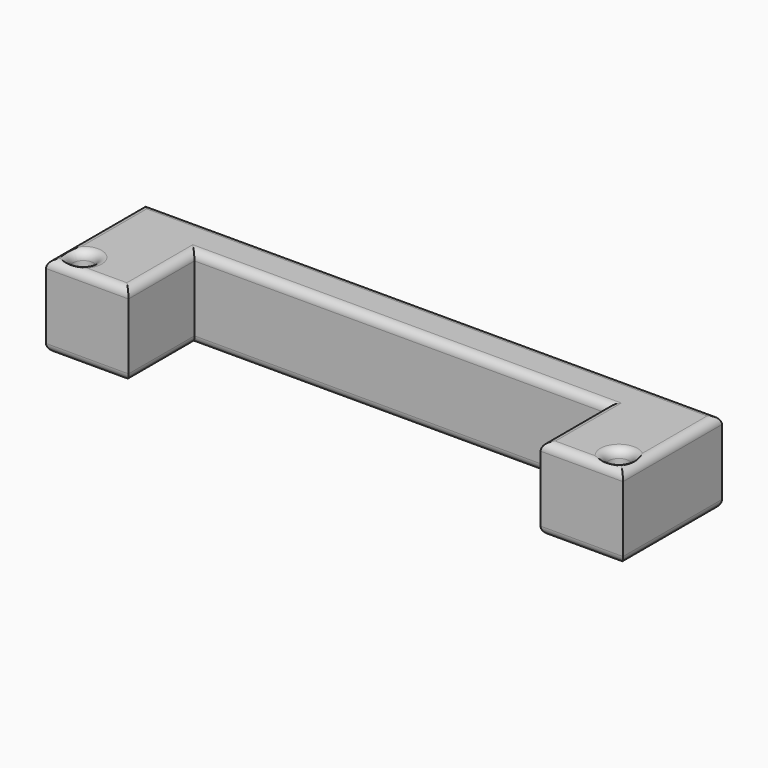
from build123d import *

# Parameters (mm, degrees)
F1_DEPTH     = 20
F3_D         = 5
F5_T1_DEPTH  = 150
F5_T3_DEPTH  = 40
F5_T5_DEPTH  = 30
F5_T7_DEPTH  = 25
F5_T9_DEPTH  = 100
F5_T11_DEPTH = 30
F5_T25_DEPTH = 105
F5_T29_DEPTH = 30
F5_T36_DEPTH = 30
F5_T40_DEPTH = 105
F5_T47_DEPTH = 30
F5_T51_DEPTH = 105
F5_T58_DEPTH = 105
F5_T62_DEPTH = 30


# Not quite as in the source:
# - a fillet or chamfer that OpenCascade refuses, or shapes differently, is made with other operations: its cross-section is extruded or revolved along the edge and cut away or added


with BuildPart() as f1:
    # F0 (on Top) → F1 (new body)
    with BuildSketch(Plane.XY):
        Polygon((70, 30), (0, 30), (0, 20), (50, 20), (50, 0), (70, 0), align=None)
    extrude(amount=F1_DEPTH)

    # F3 (through all)
    with Locations(Plane.XY.offset(20)):
        with Locations((65, 5)):
            Hole(F3_D / 2)

    # F4: F1 across face


with BuildPart() as f1_1:
    add(f1.part)
    add(f1.part.mirror(Plane(origin=(0, 25, 10), x_dir=(0, -1, 0), z_dir=(-1, 0, 0))))

    # F5: fillet of radius 2 on 20 edges, made by hand

    # F5_s2 → F5_t1 (cut)
    with BuildSketch(Plane.YZ.offset(-75)):
        with BuildLine():
            ThreePointArc((30, 18), (29.4142135624, 19.4142135624), (28, 20))
            Line((28, 20), (30, 20))
            Line((30, 20), (30, 18))
        make_face()
        with BuildLine():
            ThreePointArc((30, 2), (29.4142135624, 0.5857864376), (28, 0))
            Line((28, 0), (30, 0))
            Line((30, 0), (30, 2))
        make_face()
    extrude(amount=F5_T1_DEPTH, mode=Mode.SUBTRACT)

    # F5_s4 → F5_t3 (cut)
    with BuildSketch(Plane.XZ.offset(-35)):
        with BuildLine():
            ThreePointArc((-70, 18), (-69.4142135624, 19.4142135624), (-68, 20))
            Line((-68, 20), (-70, 20))
            Line((-70, 20), (-70, 18))
        make_face()
        with BuildLine():
            ThreePointArc((68, 20), (69.4142135624, 19.4142135624), (70, 18))
            Line((70, 18), (70, 20))
            Line((70, 20), (68, 20))
        make_face()
        with BuildLine():
            ThreePointArc((-68, 0), (-69.4142135624, 0.5857864376), (-70, 2))
            Line((-70, 2), (-70, 0))
            Line((-70, 0), (-68, 0))
        make_face()
        with BuildLine():
            ThreePointArc((68, 0), (69.4142135624, 0.5857864376), (70, 2))
            Line((70, 2), (70, 0))
            Line((70, 0), (68, 0))
        make_face()
    extrude(amount=F5_T3_DEPTH, mode=Mode.SUBTRACT)

    # F5_s6 → F5_t5 (cut)
    with BuildSketch(Plane.YZ.offset(-75)):
        with BuildLine():
            ThreePointArc((0, 18), (0.5857864376, 19.4142135624), (2, 20))
            Line((2, 20), (0, 20))
            Line((0, 20), (0, 18))
        make_face()
        with BuildLine():
            ThreePointArc((2, 0), (0.5857864376, 0.5857864376), (0, 2))
            Line((0, 2), (0, 0))
            Line((0, 0), (2, 0))
        make_face()
    extrude(amount=F5_T5_DEPTH, mode=Mode.SUBTRACT)

    # F5_s8 → F5_t7 (cut)
    with BuildSketch(Plane.XZ.offset(-20)):
        with BuildLine():
            ThreePointArc((-50, 18), (-50.5857864376, 19.4142135624), (-52, 20))
            Line((-52, 20), (-50, 20))
            Line((-50, 20), (-50, 18))
        make_face()
        with BuildLine():
            ThreePointArc((50, 18), (50.5857864376, 19.4142135624), (52, 20))
            Line((52, 20), (50, 20))
            Line((50, 20), (50, 18))
        make_face()
        with BuildLine():
            ThreePointArc((-52, 0), (-50.5857864376, 0.5857864376), (-50, 2))
            Line((-50, 2), (-50, 0))
            Line((-50, 0), (-52, 0))
        make_face()
        with BuildLine():
            ThreePointArc((52, 0), (50.5857864376, 0.5857864376), (50, 2))
            Line((50, 2), (50, 0))
            Line((50, 0), (52, 0))
        make_face()
    extrude(amount=F5_T7_DEPTH, mode=Mode.SUBTRACT)

    # F5_s10 → F5_t9 (cut)
    with BuildSketch(Plane.YZ.offset(-50)):
        with BuildLine():
            ThreePointArc((20, 18), (20.5857864376, 19.4142135624), (22, 20))
            Line((22, 20), (20, 20))
            Line((20, 20), (20, 18))
        make_face()
        with BuildLine():
            ThreePointArc((22, 0), (20.5857864376, 0.5857864376), (20, 2))
            Line((20, 2), (20, 0))
            Line((20, 0), (22, 0))
        make_face()
    extrude(amount=F5_T9_DEPTH, mode=Mode.SUBTRACT)

    # F5_s12 → F5_t11 (cut)
    with BuildSketch(Plane.YZ.offset(45)):
        with BuildLine():
            ThreePointArc((0, 18), (0.5857864376, 19.4142135624), (2, 20))
            Line((2, 20), (0, 20))
            Line((0, 20), (0, 18))
        make_face()
        with BuildLine():
            ThreePointArc((2, 0), (0.5857864376, 0.5857864376), (0, 2))
            Line((0, 2), (0, 0))
            Line((0, 0), (2, 0))
        make_face()
    extrude(amount=F5_T11_DEPTH, mode=Mode.SUBTRACT)

    # F5_s13 → F5_t14 (revolve, cut)
    with BuildSketch(Plane.XZ.offset(-5)):
        with BuildLine():
            ThreePointArc((67.5, 18), (68.0857864376, 19.4142135624), (69.5, 20))
            Line((69.5, 20), (67.5, 20))
            Line((67.5, 20), (67.5, 18))
        make_face()
    revolve(axis=Axis((65, 5, 20), (0, 0, 1)), mode=Mode.SUBTRACT)

    # F5_s15 → F5_t16 (revolve, cut)
    with BuildSketch(Plane.XZ.offset(-5)):
        with BuildLine():
            ThreePointArc((-67.5, 18), (-68.0857864376, 19.4142135624), (-69.5, 20))
            Line((-69.5, 20), (-67.5, 20))
            Line((-67.5, 20), (-67.5, 18))
        make_face()
    revolve(axis=Axis((-65, 5, 20), (0, 0, -1)), mode=Mode.SUBTRACT)

    # F5_s17 → F5_t18 (revolve, cut)
    with BuildSketch(Plane.XZ.offset(-5)):
        with BuildLine():
            ThreePointArc((69.5, 0), (68.0857864376, 0.5857864376), (67.5, 2))
            Line((67.5, 2), (67.5, 0))
            Line((67.5, 0), (69.5, 0))
        make_face()
    revolve(axis=Axis((65, 5, 0), (0, 0, 1)), mode=Mode.SUBTRACT)

    # F5_s19 → F5_t20 (revolve, cut)
    with BuildSketch(Plane.XZ.offset(-5)):
        with BuildLine():
            ThreePointArc((-69.5, 0), (-68.0857864376, 0.5857864376), (-67.5, 2))
            Line((-67.5, 2), (-67.5, 0))
            Line((-67.5, 0), (-69.5, 0))
        make_face()
    revolve(axis=Axis((-65, 5, 0), (0, 0, -1)), mode=Mode.SUBTRACT)


with BuildPart() as f5_tool23:
    # F5_s24 → F5_t25 (new body)
    with BuildSketch(Plane.YZ.offset(-55)):
        with BuildLine():
            ThreePointArc((20, 18), (20.5857864376, 19.4142135624), (22, 20))
            Line((22, 20), (20, 20))
            Line((20, 20), (20, 18))
        make_face()
    extrude(amount=F5_T25_DEPTH)

    split(bisect_by=Plane.YZ.offset(-50), keep=Keep.BOTTOM)


with BuildPart() as f5_tool27:
    # F5_s28 → F5_t29 (new body)
    with BuildSketch(Plane.XZ.offset(-25)):
        with BuildLine():
            ThreePointArc((-50, 18), (-50.5857864376, 19.4142135624), (-52, 20))
            Line((-52, 20), (-50, 20))
            Line((-50, 20), (-50, 18))
        make_face()
    extrude(amount=F5_T29_DEPTH)

    split(bisect_by=Plane.XZ.offset(-20), keep=Keep.BOTTOM)


with BuildPart() as f5_tool23_1:
    add(f5_tool23.part)

    # F5_t31: intersect F5_tool27
    add(f5_tool27.part, mode=Mode.INTERSECT)


with BuildPart() as f1_2:
    add(f1_1.part)

    # F5_t21: cut F5_tool23
    add(f5_tool23_1.part, mode=Mode.SUBTRACT)


with BuildPart() as f5_tool34:
    # F5_s35 → F5_t36 (new body)
    with BuildSketch(Plane.XZ.offset(-25)):
        with BuildLine():
            ThreePointArc((50, 18), (50.5857864376, 19.4142135624), (52, 20))
            Line((52, 20), (50, 20))
            Line((50, 20), (50, 18))
        make_face()
    extrude(amount=F5_T36_DEPTH)

    split(bisect_by=Plane.XZ.offset(-20), keep=Keep.BOTTOM)


with BuildPart() as f5_tool38:
    # F5_s39 → F5_t40 (new body)
    with BuildSketch(Plane.YZ.offset(-50)):
        with BuildLine():
            ThreePointArc((20, 18), (20.5857864376, 19.4142135624), (22, 20))
            Line((22, 20), (20, 20))
            Line((20, 20), (20, 18))
        make_face()
    extrude(amount=F5_T40_DEPTH)

    split(bisect_by=Plane.YZ.offset(50), keep=Keep.TOP)


with BuildPart() as f5_tool34_1:
    add(f5_tool34.part)

    # F5_t42: intersect F5_tool38
    add(f5_tool38.part, mode=Mode.INTERSECT)


with BuildPart() as f1_3:
    add(f1_2.part)

    # F5_t32: cut F5_tool34
    add(f5_tool34_1.part, mode=Mode.SUBTRACT)


with BuildPart() as f5_tool45:
    # F5_s46 → F5_t47 (new body)
    with BuildSketch(Plane.XZ.offset(-25)):
        with BuildLine():
            ThreePointArc((-52, 0), (-50.5857864376, 0.5857864376), (-50, 2))
            Line((-50, 2), (-50, 0))
            Line((-50, 0), (-52, 0))
        make_face()
    extrude(amount=F5_T47_DEPTH)

    split(bisect_by=Plane.XZ.offset(-20), keep=Keep.BOTTOM)


with BuildPart() as f5_tool49:
    # F5_s50 → F5_t51 (new body)
    with BuildSketch(Plane.YZ.offset(50)):
        with BuildLine():
            ThreePointArc((22, 0), (20.5857864376, 0.5857864376), (20, 2))
            Line((20, 2), (20, 0))
            Line((20, 0), (22, 0))
        make_face()
    extrude(amount=-F5_T51_DEPTH)

    split(bisect_by=Plane.YZ.offset(-50), keep=Keep.BOTTOM)


with BuildPart() as f5_tool45_1:
    add(f5_tool45.part)

    # F5_t53: intersect F5_tool49
    add(f5_tool49.part, mode=Mode.INTERSECT)


with BuildPart() as f1_4:
    add(f1_3.part)

    # F5_t43: cut F5_tool45
    add(f5_tool45_1.part, mode=Mode.SUBTRACT)


with BuildPart() as f5_tool56:
    # F5_s57 → F5_t58 (new body)
    with BuildSketch(Plane.YZ.offset(55)):
        with BuildLine():
            ThreePointArc((22, 0), (20.5857864376, 0.5857864376), (20, 2))
            Line((20, 2), (20, 0))
            Line((20, 0), (22, 0))
        make_face()
    extrude(amount=-F5_T58_DEPTH)

    split(bisect_by=Plane.YZ.offset(50), keep=Keep.TOP)


with BuildPart() as f5_tool60:
    # F5_s61 → F5_t62 (new body)
    with BuildSketch(Plane.XZ.offset(-25)):
        with BuildLine():
            ThreePointArc((52, 0), (50.5857864376, 0.5857864376), (50, 2))
            Line((50, 2), (50, 0))
            Line((50, 0), (52, 0))
        make_face()
    extrude(amount=F5_T62_DEPTH)

    split(bisect_by=Plane.XZ.offset(-20), keep=Keep.BOTTOM)


with BuildPart() as f5_tool56_1:
    add(f5_tool56.part)

    # F5_t64: intersect F5_tool60
    add(f5_tool60.part, mode=Mode.INTERSECT)


with BuildPart() as f1_5:
    add(f1_4.part)

    # F5_t54: cut F5_tool56
    add(f5_tool56_1.part, mode=Mode.SUBTRACT)


solid = f1_5.part
